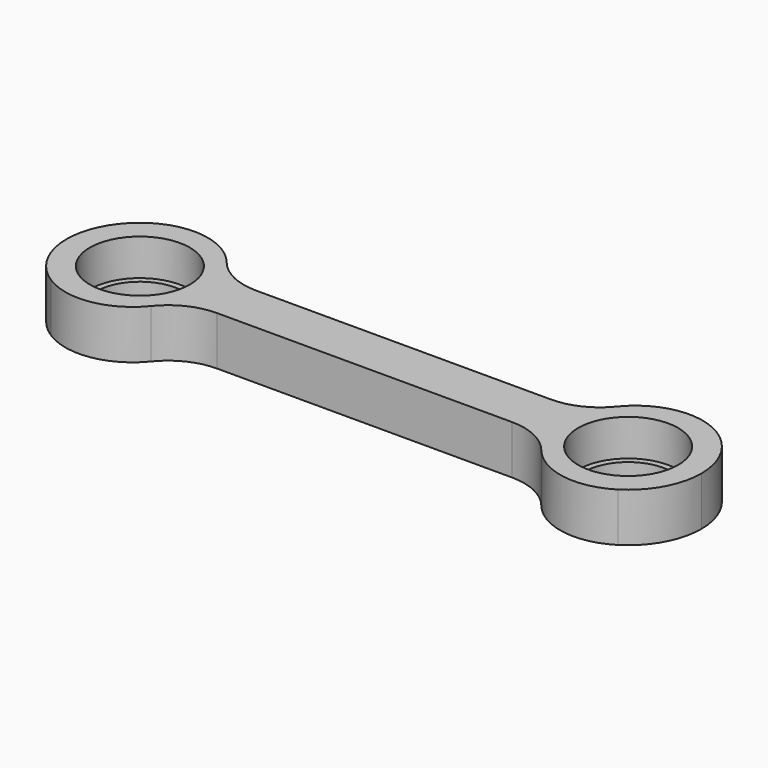
from build123d import *

# Parameters (mm, degrees)
F0_W        = 52
F0_H        = 12
F1_DEPTH    = 4
F2_R        = 4.1
F2_R_2      = 3.6
F3_DEPTH    = 3
F4_DEPTH    = 25
F5_R        = 5.99999
F6_W        = 30
F6_H        = 4
F7_DEPTH    = 25
F8_T1_DEPTH = 45.3877798739
F9_R        = 5


# Not quite as in the source:
# - a fillet or chamfer that OpenCascade refuses, or shapes differently, is made with other operations: its cross-section is extruded or revolved along the edge and cut away or added
# - a fillet or chamfer is up to 0.001 mm smaller than in the source, because OpenCascade refuses the exact size
# - a feature names something its author has since deleted; it is built from what else it names


with BuildPart() as f1:
    # F0 (on Top) → F1 (new body)
    with BuildSketch(Plane.XY):
        with Locations((6.1197612388, 6)):
            Rectangle(F0_W, F0_H)
    extrude(amount=F1_DEPTH)

    # F2 (on face) → F3 (cut)
    with BuildSketch(Plane.XY.offset(4)):
        with Locations((-13.8802387612, 6)):
            Circle(F2_R)
        with Locations((-13.8802387612, 6)):
            Circle(F2_R_2, mode=Mode.SUBTRACT)
        with Locations((26.1197612388, 6)):
            Circle(F2_R)
        with Locations((26.1197612388, 6)):
            Circle(F2_R_2, mode=Mode.SUBTRACT)
    extrude(amount=-F3_DEPTH, mode=Mode.SUBTRACT)

    # F2 (on face) → F4 (cut)
    with BuildSketch(Plane.XY.offset(4)):
        with Locations((-13.8802387612, 6)):
            Circle(F2_R_2)
        with Locations((26.1197612388, 6)):
            Circle(F2_R_2)
    extrude(amount=-F4_DEPTH, mode=Mode.SUBTRACT)

    # F5 (radius 6 in the source; OpenCascade refuses exactly that, so slightly less here)
    f5_edges = [f1.edges().sort_by_distance(p)[0] for p in [
        (32.119761, 12, 2),
        (32.119761, 0, 2),
        (-19.880239, 12, 2),
        (-19.880239, 0, 2),
    ]]
    fillet(f5_edges, radius=F5_R)

    # F6 (on face) → F7 (cut)
    with BuildSketch(Plane.XY.offset(4)):
        with Locations((6.1197612388, 10)):
            Rectangle(F6_W, F6_H)
        with Locations((6.1197612388, 2)):
            Rectangle(F6_W, F6_H)
    extrude(amount=-F7_DEPTH, mode=Mode.SUBTRACT)

    # F8: fillet of radius 5.5 on 4 edges, made by hand

    # F8_s2 → F8_t1 (cut)
    with BuildSketch(Plane.XY.offset(-20.693889937)):
        with BuildLine():
            ThreePointArc((-17.1042715454, 11.0602033843), (-12.2308229409, 11.5763851223), (-8.8802387612, 8))
            Line((-8.8802387612, 8), (-8.3533713972, 8.1578314949))
            ThreePointArc((-8.3533713972, 8.1578314949), (-8.3302387612, 10), (-8.3302387612, 12))
            Line((-8.3302387612, 12), (-8.8802387612, 12.55))
            ThreePointArc((-8.8802387612, 12.55), (-13.8802487612, 12.55), (-17.3998074599, 11.5240552176))
            Line((-17.3998074599, 11.5240552176), (-17.1042715454, 11.0602033843))
        make_face()
        with BuildLine():
            ThreePointArc((-8.8802387612, 4), (-12.2308229409, 0.4236148777), (-17.1042715454, 0.9397966157))
            Line((-17.1042715454, 0.9397966157), (-17.3998074599, 0.4759447824))
            ThreePointArc((-17.3998074599, 0.4759447824), (-13.8802487612, -0.55), (-8.8802387612, -0.55))
            Line((-8.8802387612, -0.55), (-8.3302387612, 0))
            ThreePointArc((-8.3302387612, 0), (-8.3302387612, 2), (-8.3533713972, 3.8421685051))
            Line((-8.3533713972, 3.8421685051), (-8.8802387612, 4))
        make_face()
        with BuildLine():
            ThreePointArc((29.3437940231, 0.9397966157), (24.4703454185, 0.4236148777), (21.1197612388, 4))
            Line((21.1197612388, 4), (20.5928938749, 3.8421685051))
            ThreePointArc((20.5928938749, 3.8421685051), (20.5697612388, 2), (20.5697612388, 0))
            Line((20.5697612388, 0), (21.1197612388, -0.55))
            ThreePointArc((21.1197612388, -0.55), (26.1197712388, -0.55), (29.6393299376, 0.4759447824))
            Line((29.6393299376, 0.4759447824), (29.3437940231, 0.9397966157))
        make_face()
        with BuildLine():
            ThreePointArc((21.1197612388, 8), (24.4703454185, 11.5763851223), (29.3437940231, 11.0602033843))
            Line((29.3437940231, 11.0602033843), (29.6393299376, 11.5240552176))
            ThreePointArc((29.6393299376, 11.5240552176), (26.1197712388, 12.55), (21.1197612388, 12.55))
            Line((21.1197612388, 12.55), (20.5697612388, 12))
            ThreePointArc((20.5697612388, 12), (20.5697612388, 10), (20.5928938749, 8.1578314949))
            Line((20.5928938749, 8.1578314949), (21.1197612388, 8))
        make_face()
    extrude(amount=F8_T1_DEPTH, mode=Mode.SUBTRACT)

    # F9
    f9_edges = [f1.edges().sort_by_distance(p)[0] for p in [
        (-8.880239, 8, 2),
        (-8.880239, 4, 2),
        (21.119761, 8, 2),
        (21.119761, 4, 2),
    ]]
    fillet(f9_edges, radius=F9_R)


solid = f1.part
